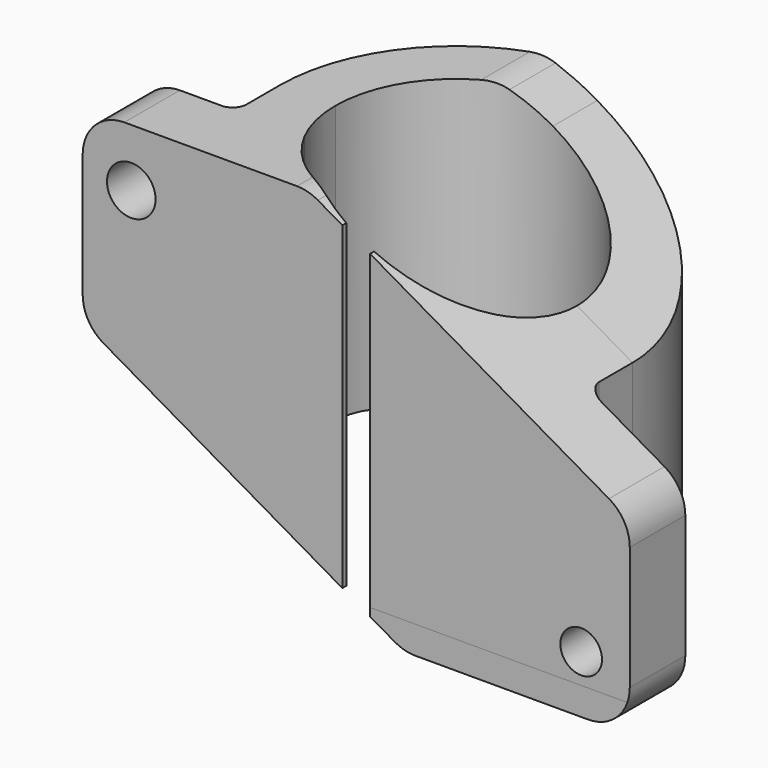
from build123d import *

# Parameters (mm, degrees)
F0_W          = 7
F0_H          = 5
F1_DEPTH      = 25
F1_DEPTH_BACK = 2
F4_DEPTH      = 25
F4_DEPTH_BACK = 25
F5_DEPTH      = 25
F5_DEPTH_BACK = 25
F6_R          = 1
F7_R          = 1.75
F7_R_2        = 1.5
F8_DEPTH      = 25
F9_T1_DEPTH   = 20
F9_T3_DEPTH   = 13.6602540378
F9_T5_DEPTH   = 8.256448117
F9_T7_DEPTH   = 5.0368572892


# Not quite as in the source:
# - a fillet or chamfer that OpenCascade refuses, or shapes differently, is made with other operations: its cross-section is extruded or revolved along the edge and cut away or added


with BuildPart() as f1:
    # F0 (on Top) → F1 (new body, two sides)
    with BuildSketch(Plane.XY) as f1_sk:
        with Locations((-16.2, -6.5)):
            Rectangle(F0_W, F0_H)
        with Locations((16.2, -6.5)):
            Rectangle(F0_W, F0_H)
        with BuildLine():
            ThreePointArc((-12.0536301586, -4), (-12.5373662109, -2.0259438524), (-12.7, 0))
            Line((-12.7, 0), (-12.7, -4))
            Line((-12.7, -4), (-12.0536301586, -4))
        make_face()
        with BuildLine():
            Line((12.7, -4), (12.7, 0))
            ThreePointArc((12.7, 0), (12.5373662109, -2.0259438524), (12.0536301586, -4))
            Line((12.0536301586, -4), (12.7, -4))
        make_face()
        with BuildLine():
            ThreePointArc((-8.7, 0), (0, 8.7), (8.7, 0))
            Line((8.7, 0), (12.7, 0))
            ThreePointArc((12.7, 0), (0, 12.7), (-12.7, 0))
            Line((-12.7, 0), (-8.7, 0))
        make_face()
        with BuildLine():
            ThreePointArc((-8.9604687377, -9), (-10.8003744429, -6.6814603115), (-12.0536301586, -4))
            Line((-12.0536301586, -4), (-12.7, -4))
            Line((-12.7, -4), (-12.7, -9))
            Line((-12.7, -9), (-8.9604687377, -9))
        make_face()
        with BuildLine():
            Line((12.7, -4), (12.0536301586, -4))
            ThreePointArc((12.0536301586, -4), (10.8003744429, -6.6814603115), (8.9604687377, -9))
            Line((8.9604687377, -9), (12.7, -9))
            Line((12.7, -9), (12.7, -4))
        make_face()
        with BuildLine():
            ThreePointArc((-7.7259303647, -4), (-8.452975635, -2.0584467235), (-8.7, 0))
            Line((-8.7, 0), (-12.7, 0))
            ThreePointArc((-12.7, 0), (-12.5373662109, -2.0259438524), (-12.0536301586, -4))
            Line((-12.0536301586, -4), (-7.7259303647, -4))
        make_face()
        with BuildLine():
            Line((12.7, 0), (8.7, 0))
            ThreePointArc((8.7, 0), (8.452975635, -2.0584467235), (7.7259303647, -4))
            Line((7.7259303647, -4), (12.0536301586, -4))
            ThreePointArc((12.0536301586, -4), (12.5373662109, -2.0259438524), (12.7, 0))
        make_face()
        with BuildLine():
            ThreePointArc((-1, -8.6423376467), (-4.9419925019, -7.1600775213), (-7.7259303647, -4))
            Line((-7.7259303647, -4), (-12.0536301586, -4))
            ThreePointArc((-12.0536301586, -4), (-10.8003744429, -6.6814603115), (-8.9604687377, -9))
            Line((-8.9604687377, -9), (-1, -9))
            Line((-1, -9), (-1, -8.6423376467))
        make_face()
        with BuildLine():
            Line((12.0536301586, -4), (7.7259303647, -4))
            ThreePointArc((7.7259303647, -4), (4.9419925019, -7.1600775213), (1, -8.6423376467))
            Line((1, -8.6423376467), (1, -9))
            Line((1, -9), (8.9604687377, -9))
            ThreePointArc((8.9604687377, -9), (10.8003744429, -6.6814603115), (12.0536301586, -4))
        make_face()
    extrude(amount=F1_DEPTH)
    extrude(f1_sk.sketch, amount=-F1_DEPTH_BACK)

    # F3 (on Front) → F4 (cut, two sides)
    with BuildSketch(Plane.XZ) as f4_sk:
        Polygon((0.0041016151, 23), (0, 23), (39.8371685741, 0), (39.8371685741, 23), (28.9984290028, 23), (28.9984290028, 6.2601172778), align=None)
        Polygon((-3.46, 25), (0.0041016151, 23), (28.9984290028, 23), (28.9984290028, 25), align=None)
        Polygon((28.9984290028, 23), (0.0041016151, 23), (28.9984290028, 6.2601172778), align=None)
    extrude(amount=F4_DEPTH, mode=Mode.SUBTRACT)
    extrude(f4_sk.sketch, amount=-F4_DEPTH_BACK, mode=Mode.SUBTRACT)

    # F2 (on Front) → F5 (cut, two sides)
    with BuildSketch(Plane.XZ) as f5_sk:
        Polygon((-0.0041016151, 0), (0, 0), (-8.2087842873, 4.739343818), (-8.2087842873, 4.7369757494), align=None)
        Polygon((3.46, -2), (-0.0041016151, 0), (-8.2087842873, 0), (-8.2087842873, 4.7369757494), (-21.54, 12.4337567297), (-21.54, -2), align=None)
        Polygon((-8.2087842873, 0), (-0.0041016151, 0), (-8.2087842873, 4.7369757494), align=None)
    extrude(amount=F5_DEPTH, mode=Mode.SUBTRACT)
    extrude(f5_sk.sketch, amount=-F5_DEPTH_BACK, mode=Mode.SUBTRACT)

    # F6
    f6_edges = [f1.edges().sort_by_distance(p)[0] for p in [
        (12.7, -4, 6.833826),
        (-12.7, -4, 16.16499),
    ]]
    fillet(f6_edges, radius=F6_R)

    # F7 (on Front) → F8 (cut)
    with BuildSketch(Plane.XZ):
        with Locations((-16.2, 20.85)):
            Circle(F7_R)
        with Locations((16.2, 2.14)):
            Circle(F7_R_2)
    extrude(amount=F8_DEPTH, mode=Mode.SUBTRACT)

    # F9: fillet of radius 3 on 8 edges, made by hand

    # F9_s2 → F9_t1 (cut)
    with BuildSketch(Plane.XZ.offset(-3.5)):
        with BuildLine():
            ThreePointArc((16.7, -2), (18.8213203436, -1.1213203436), (19.7, 1))
            Line((19.7, 1), (19.7, -2))
            Line((19.7, -2), (16.7, -2))
        make_face()
        with BuildLine():
            ThreePointArc((-19.7, 22), (-18.8213203436, 24.1213203436), (-16.7, 25))
            Line((-16.7, 25), (-19.7, 25))
            Line((-19.7, 25), (-19.7, 22))
        make_face()
    extrude(amount=F9_T1_DEPTH, mode=Mode.SUBTRACT)

    # F9_s4 → F9_t3 (cut)
    with BuildSketch(Plane.XZ.offset(-0.3301270189)):
        with BuildLine():
            ThreePointArc((18.2, 12.4922251007), (19.2980762114, 11.3941488894), (19.7, 9.8941488894))
            Line((19.7, 9.8941488894), (19.7, 11.626199697))
            Line((19.7, 11.626199697), (18.2, 12.4922251007))
        make_face()
        with BuildLine():
            ThreePointArc((-18.2, 10.5054068306), (-19.2980762114, 11.603483042), (-19.7, 13.103483042))
            Line((-19.7, 13.103483042), (-19.7, 11.3714322344))
            Line((-19.7, 11.3714322344), (-18.2, 10.5054068306))
        make_face()
    extrude(amount=F9_T3_DEPTH, mode=Mode.SUBTRACT)

    # F9_s6 → F9_t5 (cut)
    with BuildSketch(Plane.XZ.offset(-14.2292097711)):
        with BuildLine():
            ThreePointArc((-4.2638475773, 25), (-3.487390442, 24.8977774789), (-2.7638475773, 24.5980762114))
            Line((-2.7638475773, 24.5980762114), (-3.46, 25))
            Line((-3.46, 25), (-4.2638475773, 25))
        make_face()
        with BuildLine():
            ThreePointArc((4.2638475773, -2), (3.487390442, -1.8977774789), (2.7638475773, -1.5980762114))
            Line((2.7638475773, -1.5980762114), (3.46, -2))
            Line((3.46, -2), (4.2638475773, -2))
        make_face()
    extrude(amount=F9_T5_DEPTH, mode=Mode.SUBTRACT)

    # F9_s8 → F9_t7 (cut)
    with BuildSketch(Plane.XZ.offset(5.9727616541)):
        with BuildLine():
            ThreePointArc((4.2638475773, -2), (3.487390442, -1.8977774789), (2.7638475773, -1.5980762114))
            Line((2.7638475773, -1.5980762114), (3.46, -2))
            Line((3.46, -2), (4.2638475773, -2))
        make_face()
        with BuildLine():
            ThreePointArc((-4.2638475773, 25), (-3.487390442, 24.8977774789), (-2.7638475773, 24.5980762114))
            Line((-2.7638475773, 24.5980762114), (-3.46, 25))
            Line((-3.46, 25), (-4.2638475773, 25))
        make_face()
    extrude(amount=F9_T7_DEPTH, mode=Mode.SUBTRACT)


solid = f1.part
